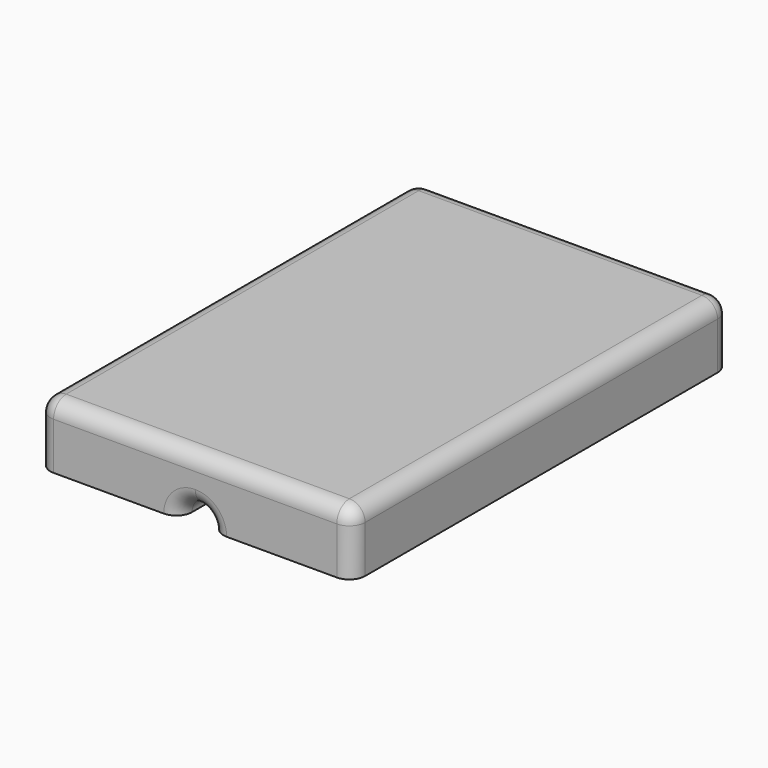
from build123d import *

# Parameters (mm, degrees)
F0_W     = 100
F0_H     = 150
F1_DEPTH = 20
F2_R     = 5
F3_D     = 5
F3_DEPTH = 12
F3_TIP   = 1.5021515476
F4_W     = 10
F4_H     = 150
F5_DEPTH = 5
F6_F1_R  = 4.9999
F6_F2_R  = 5


# Not quite as in the source:
# - a fillet or chamfer is up to 0.001 mm smaller than in the source, because OpenCascade refuses the exact size


with BuildPart() as f1:
    # F0 (on Top) → F1 (new body)
    with BuildSketch(Plane.XY):
        Rectangle(F0_W, F0_H)
    extrude(amount=F1_DEPTH)

    # F2
    f2_edges = [f1.edges().sort_by_distance(p)[0] for p in [
        (-50, 75, 10),
        (50, 75, 10),
        (0, -75, 20),
        (50, 0, 20),
        (0, 75, 20),
        (-50, 0, 20),
        (50, -75, 10),
        (-50, -75, 10),
    ]]
    fillet(f2_edges, radius=F2_R)

    # F3
    with Locations(Plane(origin=(0, 0, 0), x_dir=(1, 0, 0), z_dir=(0, 0, -1))):
        with Locations((40, -65), (-40, -65), (40, 65), (-40, 65)):
            Hole(F3_D / 2, depth=F3_DEPTH)
            with Locations((0, 0, -(F3_DEPTH + F3_TIP / 2))):  # 118° drill point
                Cone(0, F3_D / 2, F3_TIP, mode=Mode.SUBTRACT)

    # F4 (on face) → F5 (cut)
    with BuildSketch(Plane.XY):
        Rectangle(F4_W, F4_H)
    extrude(amount=F5_DEPTH, mode=Mode.SUBTRACT)

    # F6: fillet of radius 5 on 4 edges, made by hand

    # F6_f1 (radius 5 in the source; OpenCascade refuses exactly that, so slightly less here)
    f6_f1_edges = [f1.edges().sort_by_distance(p)[0] for p in [
        (5, 0, 5),
        (-5, 0, 5),
    ]]
    fillet(f6_f1_edges, radius=F6_F1_R)

    # F6_f2
    f6_f2_edges = [f1.edges().sort_by_distance(p)[0] for p in [
        (5, -75, 5e-05),
        (-5, 75, 5e-05),
        (-3.5355631953, 75, 3.5355631953),
        (3.5355631953, -75, 3.5355631953),
    ]]
    fillet(f6_f2_edges, radius=F6_F2_R)


solid = f1.part
